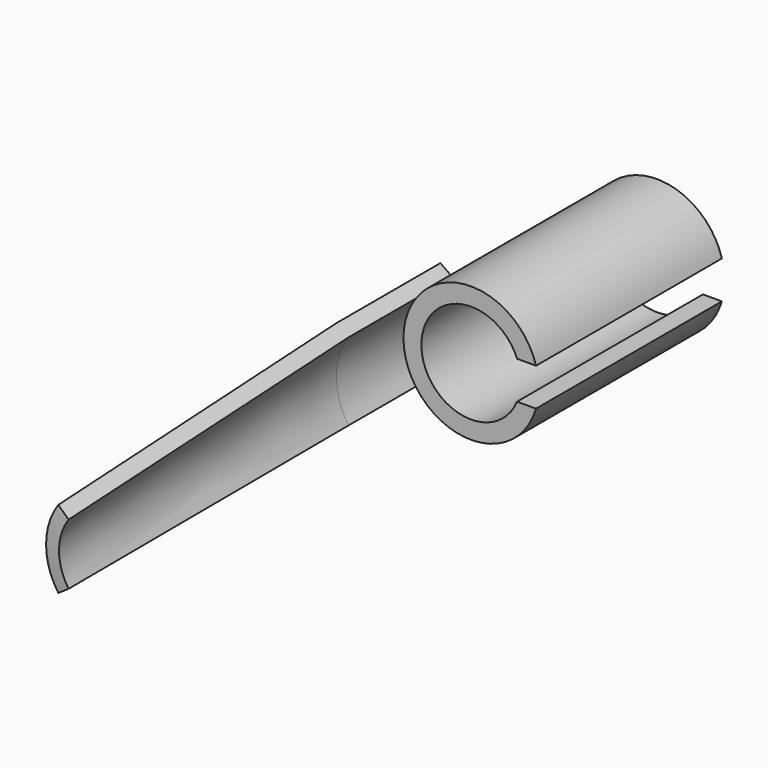
from build123d import *

# Parameters (mm, degrees)
F0_W          = 5.7658
F0_H          = 19.8156631229
F2_R          = 4.2418
F3_DEPTH      = 19.8166631229
F5_ANGLE_BACK = 35
F5_ANGLE      = 70
F7_W          = 19.842395559
F7_H          = 3.2231725054
F8_DEPTH      = 2.54


# Not quite as in the source:
# - a feature names something its author has since deleted; it is built from what else it names


with BuildPart() as f1:
    # F0 (on Top) → F1 (revolve)
    with BuildSketch(Plane.XY):
        with Locations((2.8829, 9.9078315614)):
            Rectangle(F0_W, F0_H)
    revolve(axis=Axis((5.7658, 9.9078315614, 0), (0, -1, 0)))

    # F2 (on face) → F3 (cut, through all)
    with BuildSketch(Plane(origin=(0, 19.8156631229, 0), x_dir=(-1, 0, 0), z_dir=(0, 1, 0))):
        with Locations((-5.7658, 0)):
            Circle(F2_R)
    extrude(amount=-F3_DEPTH, mode=Mode.SUBTRACT)

    # F4 (on Top) → F5 (revolve)
    with BuildSketch(Plane.XY, mode=Mode.PRIVATE) as f5_sk:
        Polygon((0, -7.1477591426), (0, 0), (0, 3.933498799), (-1.27, 3.933498799), (-1.27, 0), (-1.27, -7.1477591426), (0, -38.1), (1.2367536547, -38.268789649), align=None)
    revolve(f5_sk.sketch.rotate(Axis((5.7658, 11.3838200413, 0), (0, -1, 0)), -F5_ANGLE_BACK), axis=Axis((5.7658, 11.3838200413, 0), (0, -1, 0)), revolution_arc=F5_ANGLE)

    # F7 (on offset) → F8 (cut)
    with BuildSketch(Plane.YZ.offset(11.7856)):
        with Locations((9.9211977795, -0.010144955)):
            Rectangle(F7_W, F7_H)
    extrude(amount=-F8_DEPTH, mode=Mode.SUBTRACT)


solid = f1.part
